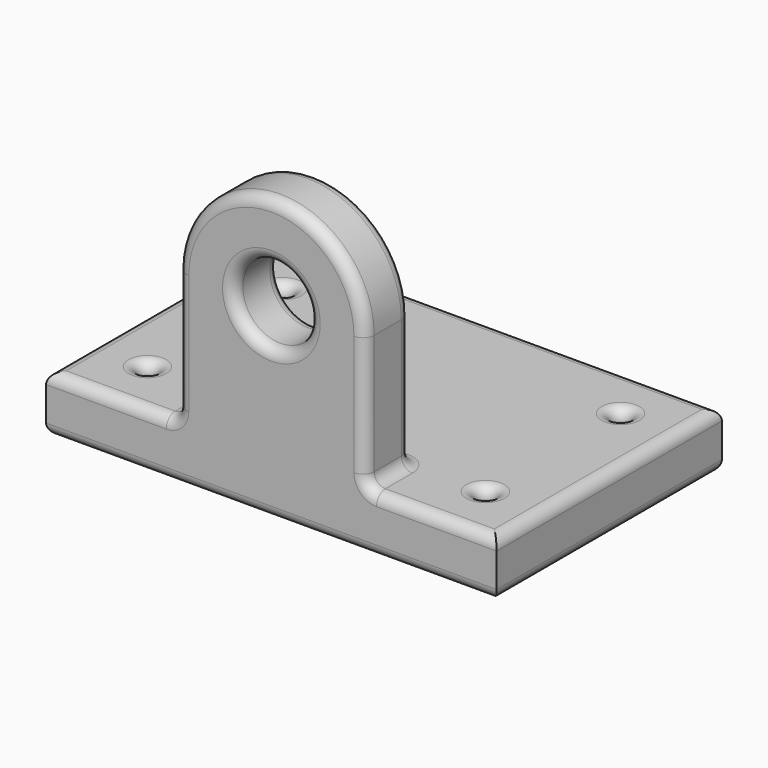
from build123d import *

# Parameters (mm, degrees)
F0_W     = 120
F0_H     = 75
F1_DEPTH = 15
F2_R     = 10
F3_DEPTH = 15
F4_R     = 2.0387597586
F5_DEPTH = 75.001
F6_R     = 3


with BuildPart() as f1:
    # F0 (on Top) → F1 (new body)
    with BuildSketch(Plane.XY):
        Rectangle(F0_W, F0_H)
    extrude(amount=F1_DEPTH)

    # F2 (on face) → F3 (join)
    with BuildSketch(Plane.XZ.offset(37.5)):
        with BuildLine():
            ThreePointArc((-25, 50), (0, 25), (25, 50))
            ThreePointArc((25, 50), (0, 75), (-25, 50))
        make_face()
        with Locations((0, 50)):
            Circle(F2_R, mode=Mode.SUBTRACT)
        with BuildLine():
            Line((25, 15), (25, 50))
            ThreePointArc((25, 50), (0, 25), (-25, 50))
            Line((-25, 50), (-25, 15))
            Line((-25, 15), (25, 15))
        make_face()
    extrude(amount=-F3_DEPTH)

    # F4 (on Top) → F5 (cut, through all)
    with BuildSketch(Plane.XY):
        with Locations((45, 22.5)):
            Circle(F4_R)
        with Locations((-45, 22.5)):
            Circle(F4_R)
        with Locations((-45, -22.5)):
            Circle(F4_R)
        with Locations((45, -22.5)):
            Circle(F4_R)
    extrude(amount=F5_DEPTH, mode=Mode.SUBTRACT)

    # F6
    f6_edges = [f1.edges().sort_by_distance(p)[0] for p in [
        (0, -37.5, 75),
        (0, -22.5, 75),
        (60, 0, 15),
        (-60, 0, 15),
        (0, 37.5, 15),
        (-42.5, -37.5, 15),
        (-47.03876, -22.5, 15),
        (-47.03876, 22.5, 15),
        (42.96124, 22.5, 15),
        (42.96124, -22.5, 15),
        (-25, -37.5, 32.5),
        (-25, -22.5, 32.5),
        (25, -22.5, 32.5),
        (25, -37.5, 32.5),
        (-10, -22.5, 50),
        (-10, -37.5, 50),
        (-25, -30, 15),
        (0, -37.5, 0),
        (-60, 0, 0),
        (60, 0, 0),
        (0, 37.5, 0),
        (-47.03876, -22.5, 0),
        (42.96124, -22.5, 0),
        (-47.03876, 22.5, 0),
        (42.96124, 22.5, 0),
        (42.5, -37.5, 15),
        (0, -22.5, 15),
        (25, -30, 15),
    ]]
    fillet(f6_edges, radius=F6_R)


solid = f1.part
